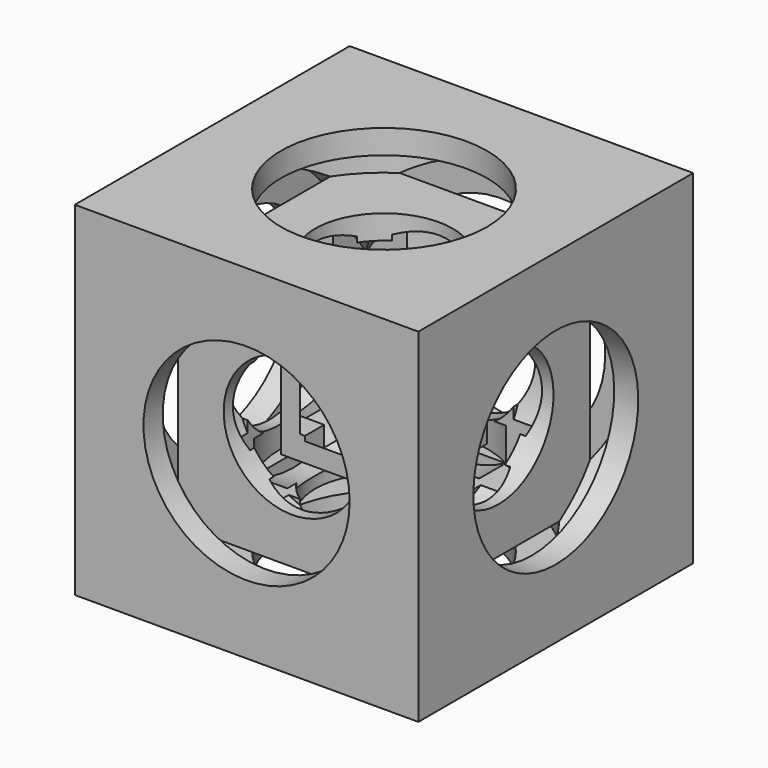
from build123d import *

# Parameters (mm, degrees)
F0_W            = 50
F0_H            = 50
F1_DEPTH        = 25
F3_COPIES_COUNT = 4


# Not quite as in the source:
# - a pattern or mirror of a feature is missing from the dataset's text; its kind, count and spacing are read off the source's solid


with BuildPart() as f1:
    # F0 (on Top) → F1 (new body, symmetric)
    with BuildSketch(Plane.XY):
        Rectangle(F0_W, F0_H)
    extrude(amount=F1_DEPTH, both=True)

    # F2 (on Front) → F3 (revolve, cut)
    with BuildSketch(Plane.XZ):
        Polygon((0, 25), (0, 0), (10, 0), (10, 4.8333333333), (5, 4.8333333333), (5, 8.3333333333), (15, 8.3333333333), (15, 13.1666666667), (10, 13.1666666667), (10, 16.6666666667), (20, 16.6666666667), (20, 21.5), (15, 21.5), (15, 25), align=None)
    f3 = revolve(axis=Axis((0, 0, 12.5), (0, 0, 1)), mode=Mode.SUBTRACT)

    # F3_copies: F3 ×4 about axis
    f3_copies_axis = Axis((0, 0, 0), (0, 1, 0))
    for i in range(1, F3_COPIES_COUNT):
        add(f3.rotate(f3_copies_axis, i * 360 / F3_COPIES_COUNT), mode=Mode.SUBTRACT)

    # F3_copies1: F3 across plane
    add(f3.mirror(Plane(origin=(0, 0, 0), x_dir=(0, -0.7071067812, 0.7071067812), z_dir=(0, -0.7071067812, -0.7071067812))), mode=Mode.SUBTRACT)

    # F3_copies2: F3 across plane
    add(f3.mirror(Plane(origin=(0, 0, 0), x_dir=(0, -0.7071067812, -0.7071067812), z_dir=(0, 0.7071067812, -0.7071067812))), mode=Mode.SUBTRACT)


solid = f1.part
